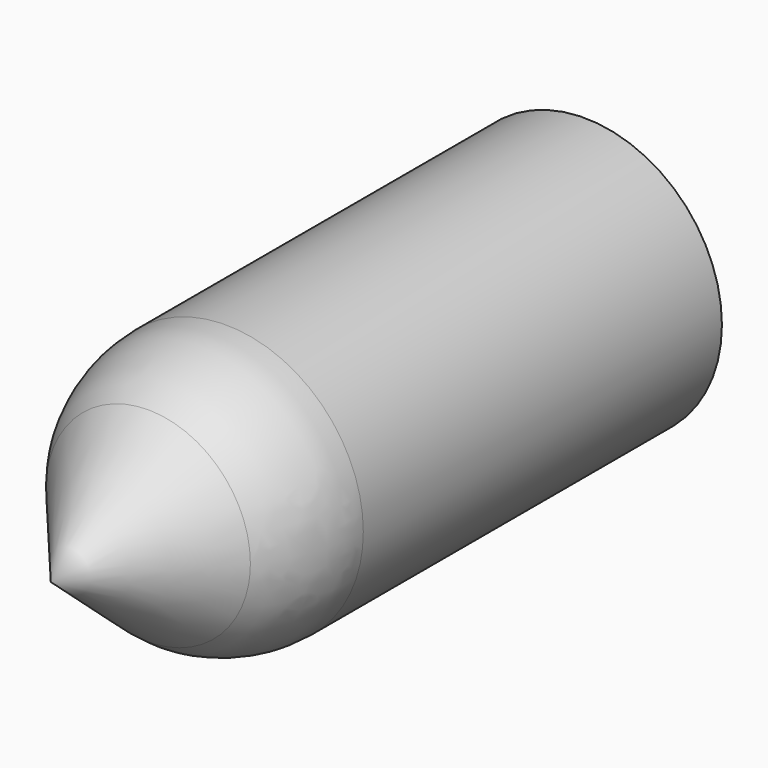
from build123d import *

# Parameters (mm, degrees)
F0_R      = 20.8202658932
F1_DEPTH  = 76.2
F1_FACE_R = 20.8202658932
F3_R      = 22.86


# Not quite as in the source:
# - an extrude whose draft closes it to a point is written as a loft to that point


with BuildPart() as f1:
    # F0 (on Front) → F1 (new body)
    with BuildSketch(Plane.XZ):
        Circle(F0_R)
    extrude(amount=F1_DEPTH)

    # F1_face (on face) → F2 section 0
    with BuildSketch(Plane.XZ.offset(76.2), mode=Mode.PRIVATE) as f2_s0:
        Circle(F1_FACE_R)
    loft([f2_s0.sketch, Vertex(0, -101.0126266769, 0)], ruled=True)

    # F3
    f3_edges = [f1.edges().sort_by_distance(p)[0] for p in [
        (-20.820266, -76.2, 0),
    ]]
    fillet(f3_edges, radius=F3_R)


solid = f1.part
